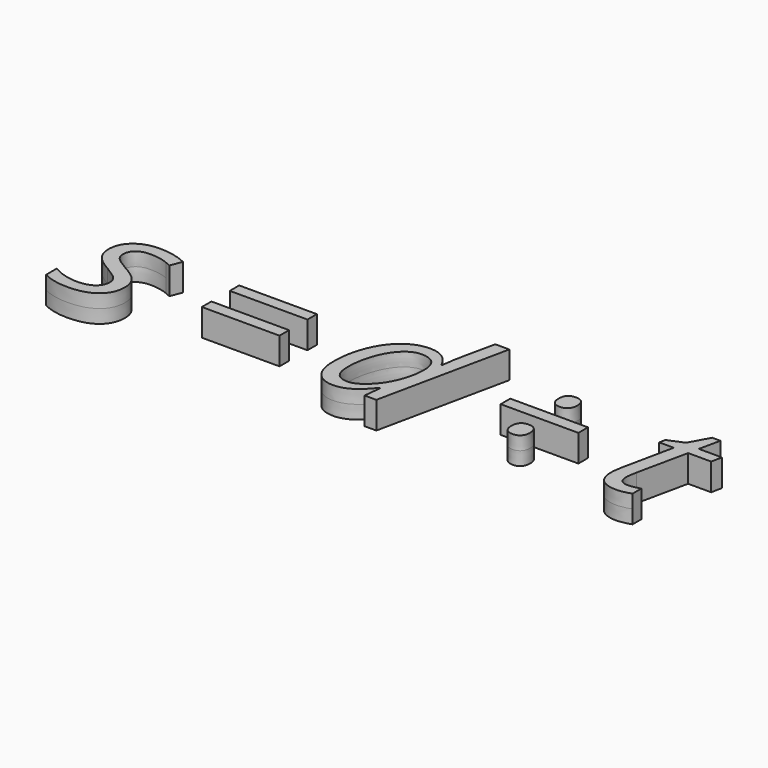
from build123d import *

# Parameters (mm, degrees)
F0_TEXT_SIZE = 40.6019356853
F1_DEPTH     = 3.175


# Not quite as in the source:
# - Text() gives the source's letters only with a copy of the font that has no kerning and outlines rounded to 1/6400 em; it was checked with that copy


with BuildPart() as f1:
    # F0 (on Top) → F1 (new body, symmetric)
    with BuildSketch(Plane.XY):
        with Locations((-69.8456078527, -13.9691215705)):
            Text('s = d ÷ t', F0_TEXT_SIZE, font='Open Sans', font_style=FontStyle.ITALIC, text_align=(TextAlign.LEFT, TextAlign.BOTTOM))
    extrude(amount=F1_DEPTH, both=True)


solid = f1.part
